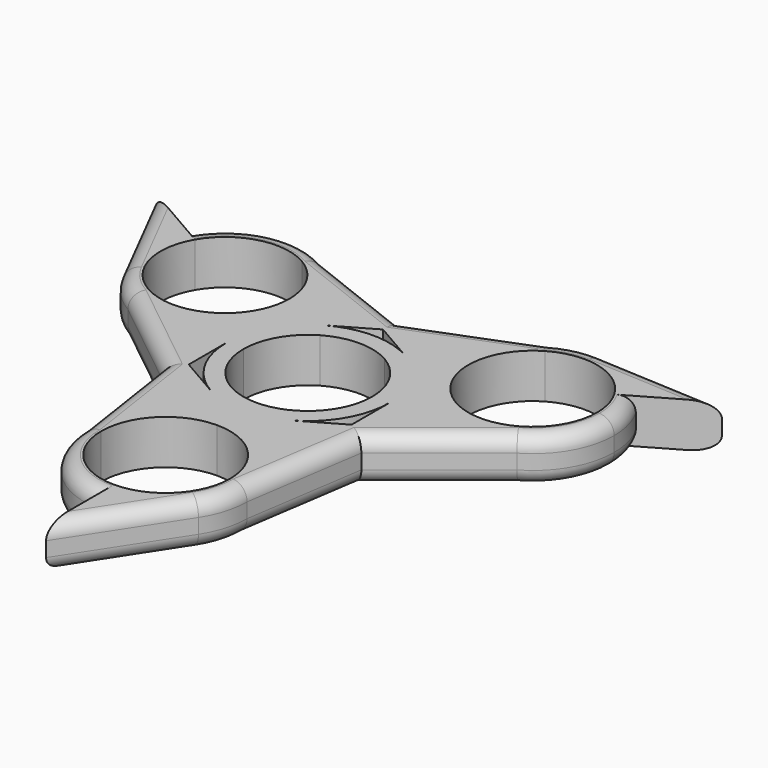
from build123d import *

# Parameters (mm, degrees)
F1_DEPTH = 7.62
F2_R     = 2.54


# Not quite as in the source:
# - a feature names something its author has since deleted; it is built from what else it names


with BuildPart() as f1:
    # F0 (on Top) → F1 (new body)
    with BuildSketch(Plane.XY):
        with BuildLine():
            Line((5.5245, 9.5687146864), (6.985, 12.0983748909))
            ThreePointArc((6.985, 12.0983748909), (0, 13.97), (-6.985, 12.0983748909))
            Line((-6.985, 12.0983748909), (-5.5245, 9.5687146864))
            ThreePointArc((-5.5245, 9.5687146864), (0, 11.049), (5.5245, 9.5687146864))
        make_face()
        with BuildLine():
            Line((0, 16.1311665212), (6.985, 12.0983748909))
            ThreePointArc((6.985, 12.0983748909), (9.8782817332, 9.8782817332), (12.0983748909, 6.985))
            Line((12.0983748909, 6.985), (14.2980794165, 8.255))
            ThreePointArc((14.2980794165, 8.255), (12.9024705141, 18.8557020601), (19.4114543073, 27.3383748909))
            Line((19.4114543073, 27.3383748909), (0, 16.1311665212))
        make_face()
        with BuildLine():
            ThreePointArc((12.0983748909, 6.985), (9.8782817332, 9.8782817332), (6.985, 12.0983748909))
            Line((6.985, 12.0983748909), (5.5245, 9.5687146864))
            ThreePointArc((5.5245, 9.5687146864), (7.8128228253, 7.8128228253), (9.5687146864, 5.5245))
            Line((9.5687146864, 5.5245), (12.0983748909, 6.985))
        make_face()
        with BuildLine():
            Line((-5.5245, 9.5687146864), (-6.985, 12.0983748909))
            ThreePointArc((-6.985, 12.0983748909), (-9.8782817332, 9.8782817332), (-12.0983748909, 6.985))
            Line((-12.0983748909, 6.985), (-9.5687146864, 5.5245))
            ThreePointArc((-9.5687146864, 5.5245), (-7.8128228253, 7.8128228253), (-5.5245, 9.5687146864))
        make_face()
        with BuildLine():
            ThreePointArc((-12.0983748909, 6.985), (-9.8782817332, 9.8782817332), (-6.985, 12.0983748909))
            Line((-6.985, 12.0983748909), (0, 16.1311665212))
            Line((0, 16.1311665212), (-19.4114543073, 27.3383748909))
            ThreePointArc((-19.4114543073, 27.3383748909), (-14.2980794165, 22.225), (-12.4264543073, 15.24))
            ThreePointArc((-12.4264543073, 15.24), (-12.9024705141, 11.6242979399), (-14.2980794165, 8.255))
            Line((-14.2980794165, 8.255), (-12.0983748909, 6.985))
        make_face()
        with BuildLine():
            Line((14.2980794165, 8.255), (12.0983748909, 6.985))
            ThreePointArc((12.0983748909, 6.985), (13.4939837933, 3.6157020601), (13.97, 0))
            Line((13.97, 0), (13.97, -8.0655832606))
            Line((13.97, -8.0655832606), (33.3814543073, 3.1416251091))
            ThreePointArc((33.3814543073, 3.1416251091), (22.7807522473, 1.7460162067), (14.2980794165, 8.255))
        make_face()
        with BuildLine():
            ThreePointArc((13.97, 0), (13.4939837933, 3.6157020601), (12.0983748909, 6.985))
            Line((12.0983748909, 6.985), (9.5687146864, 5.5245))
            ThreePointArc((9.5687146864, 5.5245), (10.6725144547, 2.8596916293), (11.049, 0))
            Line((11.049, 0), (13.97, 0))
        make_face()
        Polygon((-19.4114543073, 27.3383748909), (0, 16.1311665212), (19.4114543073, 27.3383748909), (0, 19.7183748909), align=None)
        with BuildLine():
            Line((-9.5687146864, 5.5245), (-12.0983748909, 6.985))
            ThreePointArc((-12.0983748909, 6.985), (-13.4939837933, 3.6157020601), (-13.97, 0))
            Line((-13.97, 0), (-11.049, 0))
            ThreePointArc((-11.049, 0), (-10.6725144547, 2.8596916293), (-9.5687146864, 5.5245))
        make_face()
        with BuildLine():
            ThreePointArc((-13.97, 0), (-13.4939837933, 3.6157020601), (-12.0983748909, 6.985))
            Line((-12.0983748909, 6.985), (-14.2980794165, 8.255))
            ThreePointArc((-14.2980794165, 8.255), (-22.7807522473, 1.7460162067), (-33.3814543073, 3.1416251091))
            Line((-33.3814543073, 3.1416251091), (-13.97, -8.0655832606))
            Line((-13.97, -8.0655832606), (-13.97, 0))
        make_face()
        with BuildLine():
            ThreePointArc((6.985, -12.0983748909), (12.0983748909, -6.985), (13.97, 0))
            Line((13.97, 0), (11.049, 0))
            ThreePointArc((11.049, 0), (9.5687146864, -5.5245), (5.5245, -9.5687146864))
            Line((5.5245, -9.5687146864), (6.985, -12.0983748909))
        make_face()
        with BuildLine():
            Line((16.8277396209, 9.7155), (14.2980794165, 8.255))
            ThreePointArc((14.2980794165, 8.255), (22.7807522473, 1.7460162067), (33.3814543073, 3.1416251091))
            Line((33.3814543073, 3.1416251091), (31.9209543073, 5.6712853136))
            ThreePointArc((31.9209543073, 5.6712853136), (23.536762678, 4.5674855453), (16.8277396209, 9.7155))
        make_face()
        with BuildLine():
            ThreePointArc((19.4114543073, 27.3383748909), (12.9024705141, 18.8557020601), (14.2980794165, 8.255))
            Line((14.2980794165, 8.255), (16.8277396209, 9.7155))
            ThreePointArc((16.8277396209, 9.7155), (15.7239398527, 18.0996916293), (20.8719543073, 24.8087146864))
            Line((20.8719543073, 24.8087146864), (19.4114543073, 27.3383748909))
        make_face()
        with BuildLine():
            ThreePointArc((27.1314868364, 29.1906497046), (23.137120964, 28.8244634107), (19.4114543073, 27.3383748909))
            Line((19.4114543073, 27.3383748909), (20.8719543073, 24.8087146864))
            ThreePointArc((20.8719543073, 24.8087146864), (29.2561459367, 25.9125144547), (35.9651689938, 20.7645))
            Line((35.9651689938, 20.7645), (38.4948291982, 22.225))
            ThreePointArc((38.4948291982, 22.225), (33.6974237946, 27.1503629057), (27.1314868364, 29.1906497046))
        make_face()
        with BuildLine():
            Line((-20.8719543073, 24.8087146864), (-19.4114543073, 27.3383748909))
            ThreePointArc((-19.4114543073, 27.3383748909), (-30.0121563674, 28.7339837933), (-38.4948291982, 22.225))
            Line((-38.4948291982, 22.225), (-35.9651689938, 20.7645))
            ThreePointArc((-35.9651689938, 20.7645), (-29.2561459367, 25.9125144547), (-20.8719543073, 24.8087146864))
        make_face()
        with BuildLine():
            ThreePointArc((-12.4264543073, 15.24), (-14.2980794165, 22.225), (-19.4114543073, 27.3383748909))
            Line((-19.4114543073, 27.3383748909), (-20.8719543073, 24.8087146864))
            ThreePointArc((-20.8719543073, 24.8087146864), (-16.8277396209, 20.7645), (-15.3474543073, 15.24))
            ThreePointArc((-15.3474543073, 15.24), (-15.7239398527, 12.3803083707), (-16.8277396209, 9.7155))
            Line((-16.8277396209, 9.7155), (-14.2980794165, 8.255))
            ThreePointArc((-14.2980794165, 8.255), (-12.9024705141, 11.6242979399), (-12.4264543073, 15.24))
        make_face()
        with BuildLine():
            Line((-11.049, 0), (-13.97, 0))
            ThreePointArc((-13.97, 0), (-12.0983748909, -6.985), (-6.985, -12.0983748909))
            Line((-6.985, -12.0983748909), (-5.5245, -9.5687146864))
            ThreePointArc((-5.5245, -9.5687146864), (-9.5687146864, -5.5245), (-11.049, 0))
        make_face()
        with BuildLine():
            ThreePointArc((-33.3814543073, 3.1416251091), (-22.7807522473, 1.7460162067), (-14.2980794165, 8.255))
            Line((-14.2980794165, 8.255), (-16.8277396209, 9.7155))
            ThreePointArc((-16.8277396209, 9.7155), (-23.536762678, 4.5674855453), (-31.9209543073, 5.6712853136))
            Line((-31.9209543073, 5.6712853136), (-33.3814543073, 3.1416251091))
        make_face()
        with BuildLine():
            Line((13.97, -8.0655832606), (6.985, -12.0983748909))
            ThreePointArc((6.985, -12.0983748909), (3.6157020601, -13.4939837933), (0, -13.97))
            Line((0, -13.97), (0, -16.51))
            ThreePointArc((0, -16.51), (9.8782817332, -20.6017182668), (13.97, -30.48))
            Line((13.97, -30.48), (13.97, -8.0655832606))
        make_face()
        with BuildLine():
            ThreePointArc((0, -13.97), (3.6157020601, -13.4939837933), (6.985, -12.0983748909))
            Line((6.985, -12.0983748909), (5.5245, -9.5687146864))
            ThreePointArc((5.5245, -9.5687146864), (2.8596916293, -10.6725144547), (0, -11.049))
            Line((0, -11.049), (0, -13.97))
        make_face()
        Polygon((33.3814543073, 3.1416251091), (13.97, -8.0655832606), (13.97, -30.48), (17.0766135768, -9.8591874454), align=None)
        with BuildLine():
            Line((31.9209543073, 5.6712853136), (33.3814543073, 3.1416251091))
            ThreePointArc((33.3814543073, 3.1416251091), (38.4948291982, 8.255), (40.3664543073, 15.24))
            ThreePointArc((40.3664543073, 15.24), (39.8904381006, 18.8557020601), (38.4948291982, 22.225))
            Line((38.4948291982, 22.225), (35.9651689938, 20.7645))
            ThreePointArc((35.9651689938, 20.7645), (37.068968762, 18.0996916293), (37.4454543073, 15.24))
            ThreePointArc((37.4454543073, 15.24), (35.9651689938, 9.7155), (31.9209543073, 5.6712853136))
        make_face()
        with BuildLine():
            Line((48.6004643005, 28.0594911467), (27.1314868364, 29.1906497046))
            ThreePointArc((27.1314868364, 29.1906497046), (33.6974237946, 27.1503629057), (38.4948291982, 22.225))
            Line((38.4948291982, 22.225), (48.6004643005, 28.0594911467))
        make_face()
        with BuildLine():
            Line((-35.9651689938, 20.7645), (-38.4948291982, 22.225))
            ThreePointArc((-38.4948291982, 22.225), (-40.3616158956, 15.6076435953), (-38.8455876154, 8.9012319905))
            ThreePointArc((-38.8455876154, 8.9012319905), (-36.5312780461, 5.6251028199), (-33.3814543073, 3.1416251091))
            Line((-33.3814543073, 3.1416251091), (-31.9209543073, 5.6712853136))
            ThreePointArc((-31.9209543073, 5.6712853136), (-37.068968762, 12.3803083707), (-35.9651689938, 20.7645))
        make_face()
        with BuildLine():
            ThreePointArc((-38.8455876154, 8.9012319905), (-40.3616158956, 15.6076435953), (-38.4948291982, 22.225))
            Line((-38.4948291982, 22.225), (-48.6004643005, 28.0594911467))
            Line((-48.6004643005, 28.0594911467), (-38.8455876154, 8.9012319905))
        make_face()
        with BuildLine():
            Line((0, -13.97), (0, -11.049))
            ThreePointArc((0, -11.049), (-2.8596916293, -10.6725144547), (-5.5245, -9.5687146864))
            Line((-5.5245, -9.5687146864), (-6.985, -12.0983748909))
            ThreePointArc((-6.985, -12.0983748909), (-3.6157020601, -13.4939837933), (0, -13.97))
        make_face()
        with BuildLine():
            ThreePointArc((0, -13.97), (-3.6157020601, -13.4939837933), (-6.985, -12.0983748909))
            Line((-6.985, -12.0983748909), (-13.97, -8.0655832606))
            Line((-13.97, -8.0655832606), (-13.97, -30.48))
            ThreePointArc((-13.97, -30.48), (-9.8782817332, -20.6017182668), (0, -16.51))
            Line((0, -16.51), (0, -13.97))
        make_face()
        Polygon((-13.97, -30.48), (-13.97, -8.0655832606), (-33.3814543073, 3.1416251091), (-17.0766135768, -9.8591874454), align=None)
        with BuildLine():
            Line((11.049, -30.48), (13.97, -30.48))
            ThreePointArc((13.97, -30.48), (9.8782817332, -20.6017182668), (0, -16.51))
            Line((0, -16.51), (0, -19.431))
            ThreePointArc((0, -19.431), (7.8128228253, -22.6671771747), (11.049, -30.48))
        make_face()
        with BuildLine():
            ThreePointArc((11.714100779, -38.0918816951), (13.3941570821, -34.4495662306), (13.97, -30.48))
            Line((13.97, -30.48), (11.049, -30.48))
            ThreePointArc((11.049, -30.48), (7.8128228253, -38.2928228253), (0, -41.529))
            Line((0, -41.529), (0, -44.45))
            ThreePointArc((0, -44.45), (6.664192101, -42.7580065011), (11.714100779, -38.0918816951))
        make_face()
        with BuildLine():
            Line((-11.049, -30.48), (-13.97, -30.48))
            ThreePointArc((-13.97, -30.48), (-9.8782817332, -40.3582817332), (0, -44.45))
            Line((0, -44.45), (0, -41.529))
            ThreePointArc((0, -41.529), (-7.8128228253, -38.2928228253), (-11.049, -30.48))
        make_face()
        with BuildLine():
            ThreePointArc((0, -16.51), (-9.8782817332, -20.6017182668), (-13.97, -30.48))
            Line((-13.97, -30.48), (-11.049, -30.48))
            ThreePointArc((-11.049, -30.48), (-7.8128228253, -22.6671771747), (0, -19.431))
            Line((0, -19.431), (0, -16.51))
        make_face()
        with BuildLine():
            Line((0, -56.1189822933), (11.714100779, -38.0918816951))
            ThreePointArc((11.714100779, -38.0918816951), (6.664192101, -42.7580065011), (0, -44.45))
            Line((0, -44.45), (0, -56.1189822933))
        make_face()
    extrude(amount=F1_DEPTH)

    # F2
    f2_edges = [f1.edges().sort_by_distance(p)[0] for p in [
        (15.523307, -20.169594, 7.62),
        (25.229034, -3.358781, 7.62),
        (9.705727, 23.528375, 7.62),
        (-9.705727, 23.528375, 7.62),
        (-25.229034, -3.358781, 7.62),
        (-15.523307, -20.169594, 7.62),
        (-9.878282, -40.358282, 7.62),
        (13.394157, -34.449566, 7.62),
        (39.890438, 11.624298, 7.62),
        (23.137121, 28.824463, 7.62),
        (-30.012156, 28.733984, 7.62),
        (-36.531278, 5.625103, 7.62),
        (9.705727, 23.528375, 0),
        (-9.705727, 23.528375, 0),
        (-30.012156, 28.733984, 0),
        (-36.531278, 5.625103, 0),
        (-25.229034, -3.358781, 0),
        (-15.523307, -20.169594, 0),
        (-9.878282, -40.358282, 0),
        (13.394157, -34.449566, 0),
        (15.523307, -20.169594, 0),
        (25.229034, -3.358781, 0),
        (39.890438, 11.624298, 0),
        (23.137121, 28.824463, 0),
        (-43.723026, 18.480362, 0),
        (-43.723026, 18.480362, 7.62),
        (5.85705, -47.105432, 0),
        (5.85705, -47.105432, 7.62),
        (37.865976, 28.62507, 0),
        (37.865976, 28.62507, 7.62),
    ]]
    fillet(f2_edges, radius=F2_R)


solid = f1.part
